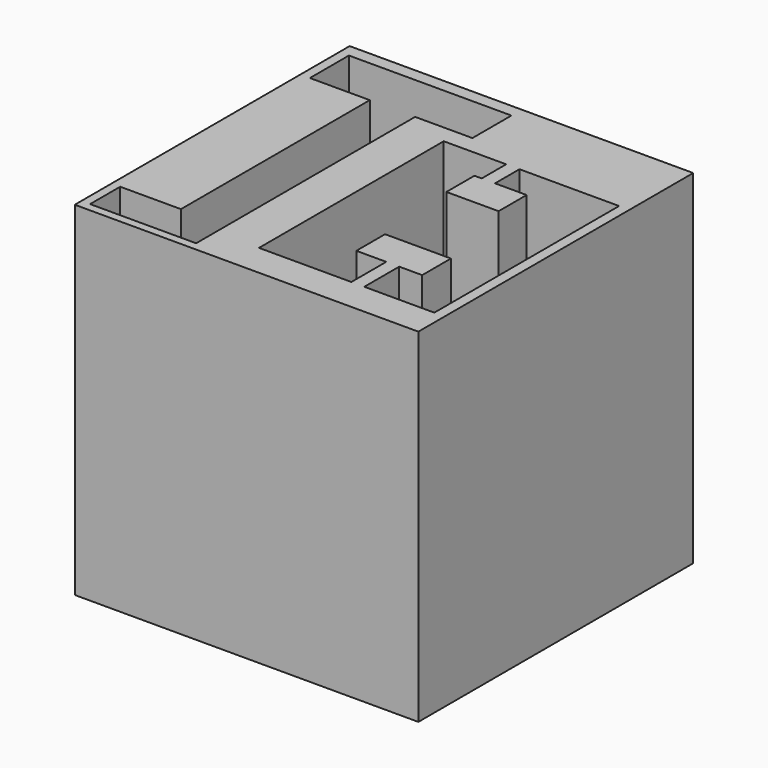
from build123d import *

# Parameters (mm, degrees)
F0_W      = 25.4
F0_H      = 25.4
F1_DEPTH  = 25.4
F2_W      = 12.0143074892
F2_H      = 3.6042919382
F3_DEPTH  = 25.401
F4_W      = 3.3513596281
F4_H      = 17.4523624592
F5_DEPTH  = 25.401
F6_W      = 7.8409165144
F6_H      = 2.7822614647
F7_DEPTH  = 25.401
F10_W     = 12.962804758
F10_H     = 17.0729630627
F11_DEPTH = 25.401
F8_W      = 3.857224714
F8_H      = 2.5925613008
F12_DEPTH = 25.4
F9_W      = 4.8689562827
F9_H      = 2.6557944948
F13_DEPTH = 25.4
F15_W     = 0.9836773388
F15_H     = 3.4875846468
F16_DEPTH = 25.4
F17_W     = 0.9571057744
F17_H     = 4.5728415716
F18_DEPTH = 25.4


with BuildPart() as f1:
    # F0 (on Top) → F1 (new body)
    with BuildSketch(Plane.XY):
        with Locations((-0.6015789695, 2.4779321572)):
            Rectangle(F0_W, F0_H)
    extrude(amount=F1_DEPTH)

    # F2 (on face) → F3 (cut, through all)
    with BuildSketch(Plane.XY.offset(25.4)):
        with Locations((-6.5916299645, 12.428777758)):
            Rectangle(F2_W, F2_H)
    extrude(amount=-F3_DEPTH, mode=Mode.SUBTRACT)

    # F4 (on face) → F5 (cut, through all)
    with BuildSketch(Plane.XY.offset(25.4)):
        with Locations((-6.4967800863, 1.9004505593)):
            Rectangle(F4_W, F4_H)
    extrude(amount=-F5_DEPTH, mode=Mode.SUBTRACT)

    # F6 (on face) → F7 (cut, through all)
    with BuildSketch(Plane.XY.offset(25.4)):
        with Locations((-8.7415585294, -8.2168614026)):
            Rectangle(F6_W, F6_H)
    extrude(amount=-F7_DEPTH, mode=Mode.SUBTRACT)

    # F10 (on face) → F11 (cut, through all)
    with BuildSketch(Plane.XY.offset(25.4)):
        with Locations((4.852715123, 0.7451490965)):
            Rectangle(F10_W, F10_H)
    extrude(amount=-F11_DEPTH, mode=Mode.SUBTRACT)



with BuildPart() as f12:
    # F8 (on face) → F12 (new body)
    with BuildSketch(Plane.XY.offset(25.4)):
        with Locations((4.3793295044, 5.7260587346)):
            Rectangle(F8_W, F8_H)
    extrude(amount=-F12_DEPTH)


with BuildPart() as f13:
    # F9 (on face) → F13 (new body)
    with BuildSketch(Plane.XY.offset(25.4)):
        with Locations((5.4218145087, -3.2385426457)):
            Rectangle(F9_W, F9_H)
    extrude(amount=-F13_DEPTH)


with BuildPart() as f1_1:
    add(f1.part)

    add(f12.part)  # F16 merges F12
    # F15 (on face) → F16 (join)
    with BuildSketch(Plane.XY):
        with Locations((3.4799792338, 8.1227321643)):
            Rectangle(F15_W, F15_H)
    extrude(amount=F16_DEPTH)


    add(f13.part)  # F18 merges F13
    # F17 (on face) → F18 (join)
    with BuildSketch(Plane.XY):
        with Locations((5.6787764188, -6.1330919852)):
            Rectangle(F17_W, F17_H)
    extrude(amount=F18_DEPTH)


solid = f1_1.part
